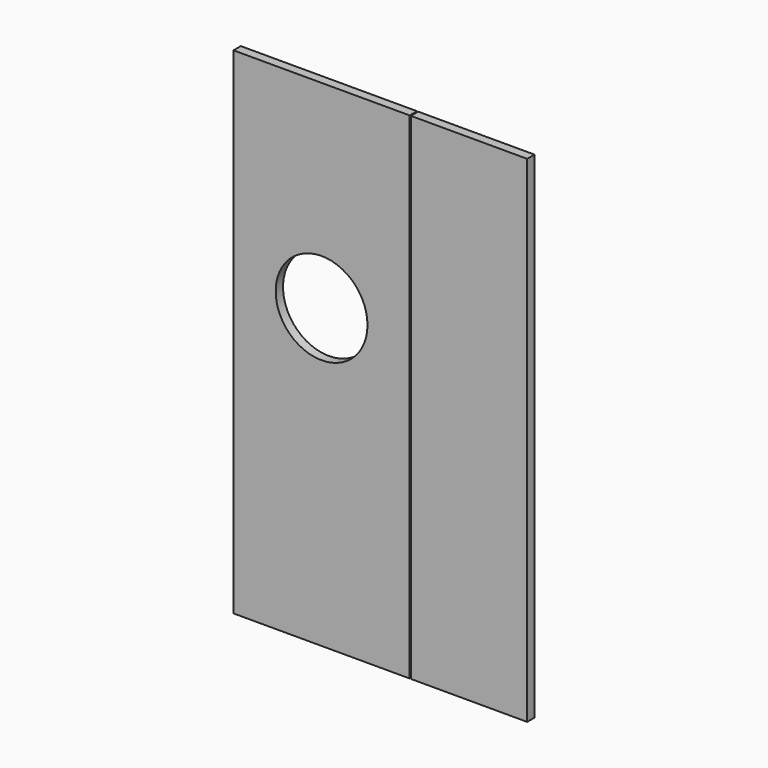
from build123d import *

# Parameters (mm, degrees)
F1_W     = 975.36
F1_H     = 50.8
F2_DEPTH = 2743.2
F1_W_2   = 643.89
F3_R     = 254
F4_DEPTH = 50.801


# Not quite as in the source:
# - a variable given as a bare number and used for a length is read in inches; the dataset says mm whatever the document's units were


with BuildPart() as f2:
    # F1 (on Top) → F2 (new body)
    with BuildSketch(Plane.XY):
        with Locations((-325.12, 25.4)):
            Rectangle(F1_W, F1_H)
    extrude(amount=F2_DEPTH)

    # F3 (on face) → F4 (cut, through all)
    with BuildSketch(Plane.XZ):
        with Locations((-325.12, 1645.92)):
            Circle(F3_R)
    extrude(amount=-F4_DEPTH, mode=Mode.SUBTRACT)


with BuildPart() as f2b:
    # F1 (on Top) → F2, piece 2 (new body)
    with BuildSketch(Plane.XY):
        with Locations((490.855, 25.4)):
            Rectangle(F1_W_2, F1_H)
    extrude(amount=F2_DEPTH)


solid = Compound([f2.part, f2b.part])
